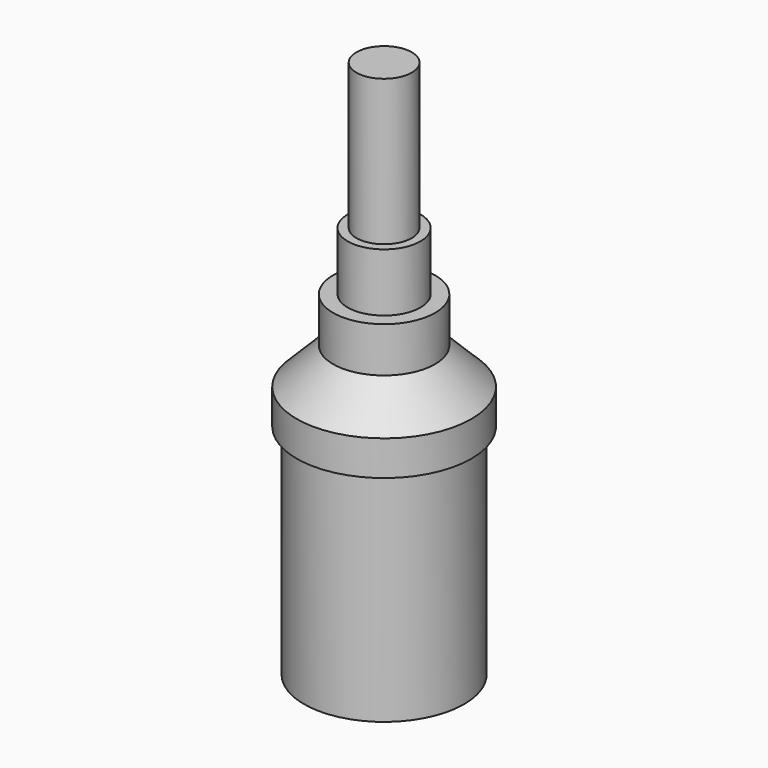
from build123d import *

# Parameters (mm, degrees)
F0_R         = 13.97
F1_DEPTH     = 38.1
F2_R         = 15.24
F3_DEPTH     = 12.7
F4_R         = 8.89
F5_DEPTH     = 7.62
F6_R         = 6.35
F7_DEPTH     = 10.16
F8_R         = 4.826
F9_DEPTH     = 25.4
F10_S5_R     = 8.89
F10_T6_DEPTH = 23
F12_D        = 20.32
F12_DEPTH    = 7.62
F12_TIP      = 6.1047438893


# Not quite as in the source:
# - a fillet or chamfer that OpenCascade refuses, or shapes differently, is made with other operations: its cross-section is extruded or revolved along the edge and cut away or added


with BuildPart() as f1:
    # F0 (on Top) → F1 (new body)
    with BuildSketch(Plane.XY):
        Circle(F0_R)
    extrude(amount=F1_DEPTH)

    # F2 (on face) → F3 (join)
    with BuildSketch(Plane.XY.offset(38.1)):
        Circle(F2_R)
    extrude(amount=F3_DEPTH)

    # F4 (on face) → F5 (join)
    with BuildSketch(Plane.XY.offset(50.8)):
        Circle(F4_R)
    extrude(amount=F5_DEPTH)

    # F6 (on face) → F7 (join)
    with BuildSketch(Plane.XY.offset(58.42)):
        Circle(F6_R)
    extrude(amount=F7_DEPTH)

    # F8 (on face) → F9 (join)
    with BuildSketch(Plane.XY.offset(68.58)):
        Circle(F8_R)
    extrude(amount=F9_DEPTH)

    # F10: chamfer of 6.604 on 1 edges, made by hand


with BuildPart() as f10_tool2:
    # F10_s3 → F10_t4 (revolve)
    with BuildSketch(Plane.XZ):
        Polygon((15.24, 44.196), (8.636, 50.8), (15.24, 50.8), align=None)
    revolve(axis=Axis((0, 0, 50.8), (0, 0, 1)))

    # F10_s5 → F10_t6 (cut, symmetric)
    with BuildSketch(Plane.XY.offset(47.5)):
        Circle(F10_S5_R)
    extrude(amount=F10_T6_DEPTH, both=True, mode=Mode.SUBTRACT)


with BuildPart() as f1_1:
    add(f1.part)

    # F10_t1: cut F10_tool2
    add(f10_tool2.part, mode=Mode.SUBTRACT)

    # F12
    with Locations(Plane(origin=(0, 0, 0), x_dir=(1, 0, 0), z_dir=(0, 0, -1))):
        with Locations((0, 0)):
            Hole(F12_D / 2, depth=F12_DEPTH)
            with Locations((0, 0, -(F12_DEPTH + F12_TIP / 2))):  # 118° drill point
                Cone(0, F12_D / 2, F12_TIP, mode=Mode.SUBTRACT)


solid = f1_1.part
